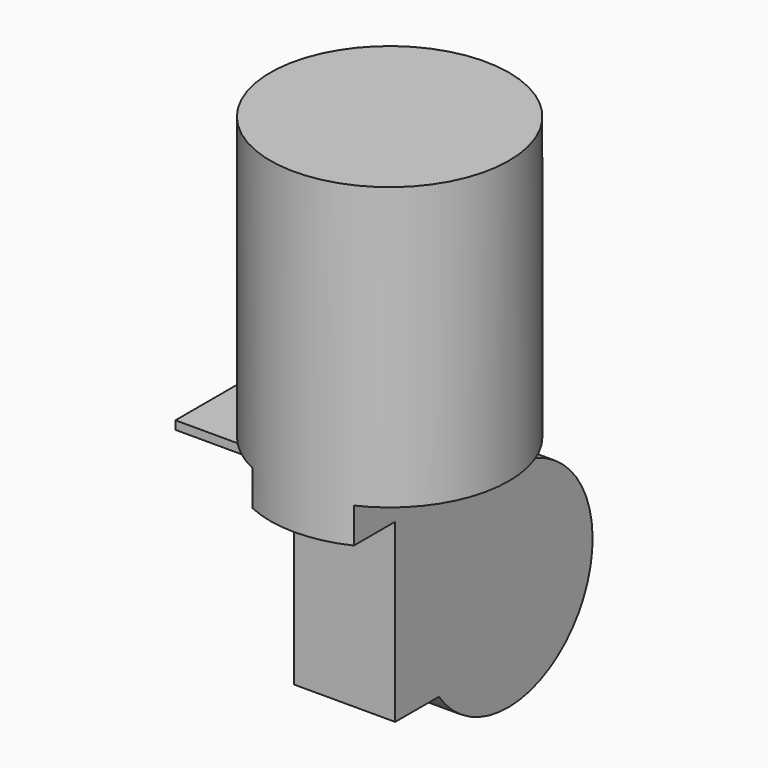
from build123d import *

# Parameters (mm, degrees)
F0_R          = 21.5
F1_DEPTH      = 57.15
F2_W          = 17.9596467465
F2_H          = 6.35
F2_W_2        = 17.1457676739
F3_DEPTH      = 21.501
F3_DEPTH_BACK = 21.501
F5_DEPTH      = 18.25
F6_W          = 28.575
F6_H          = 1.524
F7_DEPTH      = 6.35
F7_DEPTH_BACK = 23.368


with BuildPart() as f1:
    # F0 (on Top) → F1 (new body)
    with BuildSketch(Plane.XY):
        Circle(F0_R)
    extrude(amount=F1_DEPTH)

    # F2 (on Front) → F3 (cut, two sides)
    with BuildSketch(Plane.XZ) as f3_sk:
        with Locations((-18.1048233733, 3.175)):
            Rectangle(F2_W, F2_H)
        with Locations((17.6978838369, 3.175)):
            Rectangle(F2_W_2, F2_H)
    extrude(amount=-F3_DEPTH, mode=Mode.SUBTRACT)
    extrude(f3_sk.sketch, amount=F3_DEPTH_BACK, mode=Mode.SUBTRACT)

    # F4 (on face) → F5 (join, through all)
    with BuildSketch(Plane(origin=(-9.125, 0, 0), x_dir=(0, -1, 0), z_dir=(-1, 0, 0))):
        with BuildLine():
            Line((-21.5, 0), (-21.5, -2.7665854228))
            ThreePointArc((-21.5, -2.7665854228), (-30.4593629233, -32.216128711), (0.3193392569, -31.75))
            Line((0.3193392569, -31.75), (10.16, -31.75))
            Line((10.16, -31.75), (10.16, 0))
            Line((10.16, 0), (-19.4675210286, 0))
            Line((-19.4675210286, 0), (-21.5, 0))
        make_face()
    extrude(amount=-F5_DEPTH)

    # F6 (on face) → F7 (join, two sides)
    with BuildSketch(Plane(origin=(-9.125, 0, 0), x_dir=(0, -1, 0), z_dir=(-1, 0, 0))) as f7_sk:
        with Locations((-6.6675, 0.762)):
            Rectangle(F6_W, F6_H)
    extrude(amount=-F7_DEPTH)
    extrude(f7_sk.sketch, amount=F7_DEPTH_BACK)


solid = f1.part
